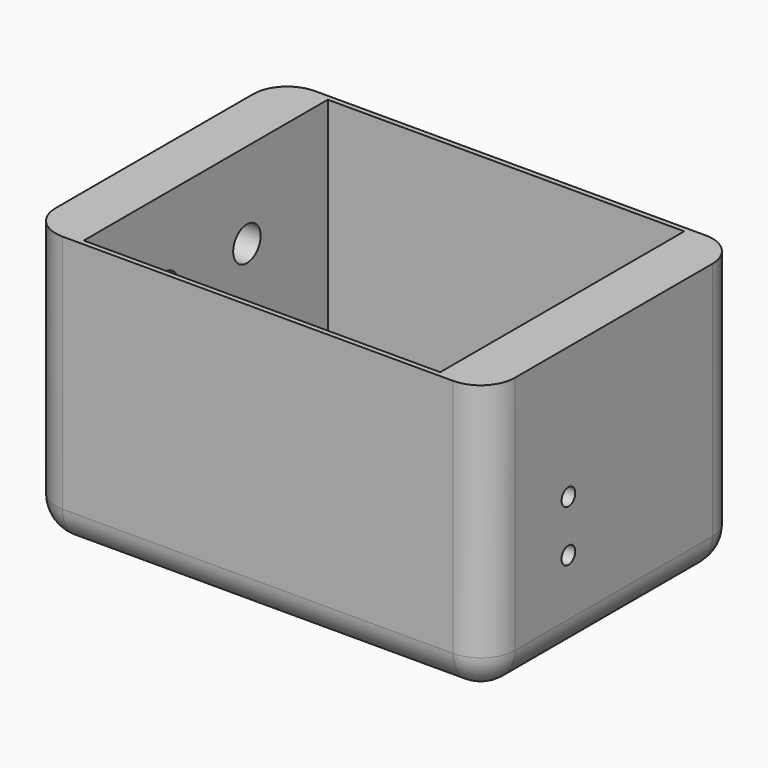
from build123d import *

# Parameters (mm, degrees)
F0_R      = 25.5
F1_DEPTH  = 2
F0_W      = 200
F0_H      = 170
F0_R_2    = 5
F2_DEPTH  = 5
F0_W_2    = 268
F0_H_2    = 184
F0_W_3    = 208
F0_H_3    = 178
F3_DEPTH  = 160
F4_DEPTH  = 40
F5_R      = 5
F6_DEPTH  = 30.3
F7_DEPTH  = 30
F8_DEPTH  = 10
F9_R      = 10
F10_DEPTH = 30
F11_R     = 20


# Not quite as in the source:
# - a feature names something its author has since deleted; it is built from what else it names


with BuildPart() as f1:
    # F0 (on Top) → F1 (new body)
    with BuildSketch(Plane.XY):
        Circle(F0_R)
    extrude(amount=F1_DEPTH)

    # F0 (on Top) → F2 (join)
    with BuildSketch(Plane.XY):
        with Locations((0, 33)):
            Rectangle(F0_W, F0_H)
        with Locations((-94, 0)):
            Circle(F0_R_2, mode=Mode.SUBTRACT)
        Circle(F0_R, mode=Mode.SUBTRACT)
        with BuildLine():
            Line((94, 10), (94, 0))
            Line((94, 0), (94, -10))
            ThreePointArc((94, -10), (90, -14), (86, -10))
            Line((86, -10), (86, 10))
            ThreePointArc((86, 10), (90, 14), (94, 10))
        make_face(mode=Mode.SUBTRACT)
    extrude(amount=F2_DEPTH)



with BuildPart() as f3:
    # F0 (on Top) → F3 (new body)
    with BuildSketch(Plane.XY):
        with Locations((0, 33)):
            Rectangle(F0_W_2, F0_H_2)
        with Locations((0, 33)):
            Rectangle(F0_W_3, F0_H_3, mode=Mode.SUBTRACT)
    extrude(amount=F3_DEPTH)


with BuildPart() as f1_1:
    add(f1.part)

    add(f3.part)  # F4 merges F3
    # F0 (on Top) → F4 (join)
    with BuildSketch(Plane.XY):
        with Locations((0, 33)):
            Rectangle(F0_W_3, F0_H_3)
        with Locations((0, 33)):
            Rectangle(F0_W, F0_H, mode=Mode.SUBTRACT)
    extrude(amount=F4_DEPTH)

    # F5 (on face) → F6 (cut)
    with BuildSketch(Plane.YZ.offset(134)):
        with Locations((0, 83)):
            Circle(F5_R)
    extrude(amount=-F6_DEPTH, mode=Mode.SUBTRACT)

    # F5 (on face) → F7 (cut)
    with BuildSketch(Plane.YZ.offset(134)):
        with Locations((0, 53)):
            Circle(F5_R)
    extrude(amount=-F7_DEPTH, mode=Mode.SUBTRACT)

    # F0 (on Top) → F8 (cut)
    with BuildSketch(Plane.XY):
        with BuildLine():
            Line((94, -10), (94, 0))
            Line((94, 0), (94, 10))
            ThreePointArc((94, 10), (90, 14), (86, 10))
            Line((86, 10), (86, -10))
            ThreePointArc((86, -10), (90, -14), (94, -10))
        make_face()
    extrude(amount=F8_DEPTH, mode=Mode.SUBTRACT)

    # F9 (on face) → F10 (cut, through all)
    with BuildSketch(Plane(origin=(-134, 0, 0), x_dir=(0, -1, 0), z_dir=(-1, 0, 0))):
        with Locations((-63, 110)):
            Circle(F9_R)
        with Locations((-3, 110)):
            Circle(F9_R)
        with Locations((-63, 50)):
            Circle(F9_R)
        with Locations((-3, 50)):
            Circle(F9_R)
    extrude(amount=-F10_DEPTH, mode=Mode.SUBTRACT)

    # F11
    f11_edges = [f1_1.edges().sort_by_distance(p)[0] for p in [
        (-134, -59, 80),
        (-134, 125, 80),
        (134, 33, 0),
        (134, -59, 80),
        (0, -59, 0),
        (0, 125, 0),
        (-134, 33, 0),
        (134, 125, 80),
    ]]
    fillet(f11_edges, radius=F11_R)


solid = f1_1.part
